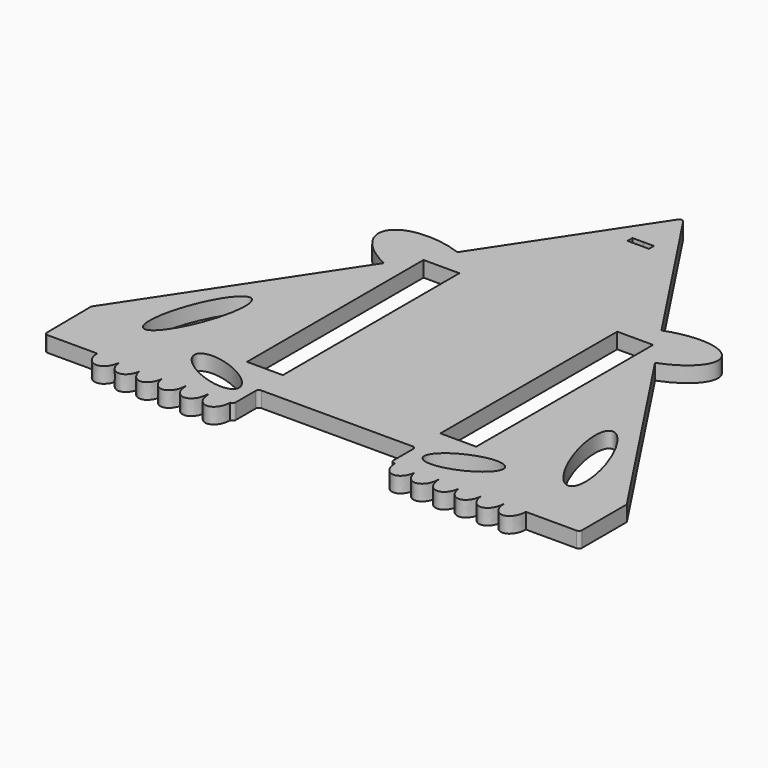
from build123d import *

# Parameters (mm, degrees)
F0_W     = 11.5
F0_H     = 70.714853704
F1_DEPTH = 5


# Not quite as in the source:
# - a feature names something its author has since deleted; it is built from what else it names


with BuildPart() as f1:
    # F0 (on Top) → F1 (new body)
    with BuildSketch(Plane.XY):
        with BuildLine():
            ThreePointArc((-85.7462971022, -48.5098765992), (-85.4499532823, -49.2105923474), (-84.7463458428, -49.5000034571))
            Line((-84.7463458428, -49.5000034571), (-68.8420371116, -49.5000034571))
            Line((-68.8420371116, -49.5000034571), (-61.4353581368, -49.5000034571))
            Line((-61.4353581368, -49.5000034571), (-54.4939316693, -49.5000034571))
            Line((-54.4939316693, -49.5000034571), (-54.4964335859, -50.4300000917))
            add(Edge.make_bspline(
                [(-54.4964335859, -50.4300000917), (-53.9357009598, -54.6615650958), (-50.9232183939, -54.4963216982), (-47.9107358281, -54.3310783007), (-47.5787906349, -50.0505473316)],
                knots=[4.89947782, 4.89947782, 4.89947782, 6.3215634822, 6.3215634822, 7.7436491443, 7.7436491443, 7.7436491443], degree=2, weights=[1, 0.7576817112, 1, 0.7576817112, 1]))
            Line((-47.5787906349, -50.0505473316), (-47.5787906349, -49.5000034571))
            Line((-47.5787906349, -49.5000034571), (-40.6000722349, -49.5000034571))
            Line((-40.6000722349, -49.5000034571), (-40.488735199, -49.5000034571))
            Line((-40.488735199, -49.5000034571), (-33.488735199, -49.5000034571))
            Line((-33.488735199, -49.5000034571), (-33.2292470932, -49.5000034571))
            Line((-33.2292470932, -49.5000034571), (-26.2365209625, -49.5000034571))
            ThreePointArc((-26.2365209625, -49.5000034571), (-26.2328840038, -49.4999968433), (-26.2292470932, -49.4999770021))
            ThreePointArc((-26.2292470932, -49.4999770021), (-25.5268471398, -49.2045338435), (-25.2365209625, -48.5000034571))
            Line((-25.2365209625, -48.5000034571), (-25.2365209625, -40.5000034571))
            ThreePointArc((-25.2365209625, -40.5000034571), (-24.9436277437, -39.7928966759), (-24.2365209625, -39.5000034571))
            Line((-24.2365209625, -39.5000034571), (24.2365209625, -39.5000034571))
            ThreePointArc((24.2365209625, -39.5000034571), (24.9436277437, -39.7928966759), (25.2365209625, -40.5000034571))
            Line((25.2365209625, -40.5000034571), (25.2365209625, -48.5000034571))
            ThreePointArc((25.2365209625, -48.5000034571), (25.5294141813, -49.2071102383), (26.2365209625, -49.5000034571))
            Line((26.2365209625, -49.5000034571), (26.6061850041, -49.5000034571))
            Line((26.6061850041, -49.5000034571), (33.528003484, -49.5000034571))
            Line((33.528003484, -49.5000034571), (33.6061850041, -49.5000034571))
            Line((33.6061850041, -49.5000034571), (40.528003484, -49.5000034571))
            Line((40.528003484, -49.5000034571), (40.6009402275, -49.5000034571))
            Line((40.6009402275, -49.5000034571), (47.5243214667, -49.5000034571))
            Line((47.5243214667, -49.5000034571), (47.6009402275, -49.5000034571))
            Line((47.6009402275, -49.5000034571), (54.5002851784, -49.5000034571))
            Line((54.5002851784, -49.5000034571), (54.5243214667, -49.5000034571))
            Line((54.5243214667, -49.5000034571), (61.5002851784, -49.5000034571))
            Line((61.5002851784, -49.5000034571), (61.5318711996, -49.5000034571))
            Line((61.5318711996, -49.5000034571), (68.5318711996, -49.5000034571))
            Line((68.5318711996, -49.5000034571), (84.7365209625, -49.5000034571))
            ThreePointArc((84.7365209625, -49.5000034571), (85.4436277437, -49.2071102383), (85.7365209625, -48.5000034571))
            Line((85.7365209625, -48.5000034571), (85.7365209625, -30.5649004877))
            Line((85.7365209625, -30.5649004877), (43.3442490508, 33.7225185076))
            Line((43.3442490508, 33.7225185076), (43.3179996887, 33.7225187957))
            add(Edge.make_bspline(
                [(43.3179996887, 33.7225187957), (58.9620766824, 39.6368972474), (54.1362258759, 47.0005661719), (49.3103750694, 54.3642350964), (33.6645006532, 48.4525992955)],
                knots=[1.7240567735, 1.7240567735, 1.7240567735, 3.2946668718, 3.2946668718, 4.86527697, 4.86527697, 4.86527697], degree=2, weights=[1, 0.7071726199, 1, 0.7071726199, 1]))
            Line((33.6645006532, 48.4525992955), (33.6018878615, 48.4967032242))
            Line((33.6018878615, 48.4967032242), (0.951977139, 98.0099375029))
            ThreePointArc((0.951977139, 98.0099375029), (0.1182843378, 98.4594332204), (-0.7164311162, 98.0118394339))
            Line((-0.7164311162, 98.0118394339), (-32.7268251846, 49.708416028))
            add(Edge.make_bspline(
                [(-32.7268251846, 49.708416028), (-48.7950217032, 55.5805403021), (-53.7532185506, 48.0986617244), (-58.7114153979, 40.6167831466), (-43.4232254677, 33.5676352963)],
                knots=[1.511873297, 1.511873297, 1.511873297, 3.0039299939, 3.0039299939, 4.4959866908, 4.4959866908, 4.4959866908], degree=2, weights=[1, 0.7343903226, 1, 0.7343903226, 1]))
            Line((-43.4232254677, 33.5676352963), (-85.9234790375, -30.5649004876))
            Line((-85.9234790375, -30.5649004876), (-85.7462971022, -48.5098765992))
        make_face()
        with BuildLine():
            add(Edge.make_bspline(
                [(-68.1659526923, -31.7135490477), (-60.5147940439, -34.4461020139), (-56.3683340858, -10.7580853655), (-52.2218741276, 12.929931283), (-64.0194927341, -8.0255323992), (-75.8171113406, -28.9809960815), (-68.1659526923, -31.7135490477)],
                knots=[0, 0, 0, 2.0943951024, 2.0943951024, 4.1887902048, 4.1887902048, 6.2831853072, 6.2831853072, 6.2831853072], degree=2, weights=[1, 0.5, 1, 0.5, 1, 0.5, 1]))
        make_face(mode=Mode.SUBTRACT)
        with BuildLine():
            add(Edge.make_bspline(
                [(-49.2456242242, -34.0520180762), (-52.2540837889, -40.9714753387), (-36.0812831751, -43.8893859564), (-19.9084825613, -46.8072965741), (-33.0728236104, -36.9699286939), (-46.2371646594, -27.1325608136), (-49.2456242242, -34.0520180762)],
                knots=[0, 0, 0, 2.0943951024, 2.0943951024, 4.1887902048, 4.1887902048, 6.2831853072, 6.2831853072, 6.2831853072], degree=2, weights=[1, 0.5, 1, 0.5, 1, 0.5, 1]))
        make_face(mode=Mode.SUBTRACT)
        with Locations((-30.9865209625, 5.7290308177)):
            Rectangle(F0_W, F0_H, mode=Mode.SUBTRACT)
        with BuildLine():
            add(Edge.make_bspline(
                [(49.4799129665, -34.0520180762), (46.4714534017, -27.1325608136), (33.3071123527, -36.9699286939), (20.1427713037, -46.8072965741), (36.3155719175, -43.8893859564), (52.4883725313, -40.9714753387), (49.4799129665, -34.0520180762)],
                knots=[0, 0, 0, 2.0943951024, 2.0943951024, 4.1887902048, 4.1887902048, 6.2831853072, 6.2831853072, 6.2831853072], degree=2, weights=[1, 0.5, 1, 0.5, 1, 0.5, 1]))
        make_face(mode=Mode.SUBTRACT)
        with BuildLine():
            add(Edge.make_bspline(
                [(68.4002414346, -31.7135490477), (76.0514000829, -28.9809960815), (64.2537814764, -8.0255323992), (52.4561628699, 12.929931283), (56.6026228281, -10.7580853655), (60.7490827862, -34.4461020139), (68.4002414346, -31.7135490477)],
                knots=[0, 0, 0, 2.0943951024, 2.0943951024, 4.1887902048, 4.1887902048, 6.2831853072, 6.2831853072, 6.2831853072], degree=2, weights=[1, 0.5, 1, 0.5, 1, 0.5, 1]))
        make_face(mode=Mode.SUBTRACT)
        Polygon((36.7681543864, -29.6869881133), (25.2681690006, -29.6686543549), (25.3809054394, 41.0461094846), (36.8808908252, 41.0277757262), align=None, mode=Mode.SUBTRACT)
        with BuildLine():
            Line((-33.5298201198, 48.4967032242), (-32.7268251846, 49.708416028))
            add(Edge.make_bspline(
                [(-31.3512903, 49.1735135083), (-32.0315452267, 49.454325887), (-32.7268251846, 49.708416028)],
                knots=[1.4319341267, 1.4319341267, 1.4319341267, 1.511873297, 1.511873297, 1.511873297], degree=2, weights=[1, 0.9992013225, 1]))
            Line((-31.3512903, 49.1735135083), (-33.5298201198, 48.4967032242))
        make_face(mode=Mode.SUBTRACT)
        Polygon((-3.3304034732, 81.0417085886), (-3.3304034732, 83.0417085886), (0, 83.0417085886), (0.211303281, 83.0415401544), (3.541702522, 83.0362306925), (3.5385140423, 81.0362332341), (0.208110569, 81.0388879667), (0, 81.0390538559), align=None, mode=Mode.SUBTRACT)
        with BuildLine():
            Line((-61.4353581368, -49.5000034571), (-68.8420371116, -49.5000034571))
            add(Edge.make_bspline(
                [(-68.8420371116, -49.5000034571), (-68.8420371116, -54.5000034571), (-65.1386976242, -54.5000034571), (-61.4353581368, -54.5000034571), (-61.4353581368, -49.5000034571)],
                knots=[4.7123889804, 4.7123889804, 4.7123889804, 6.2831853072, 6.2831853072, 7.853981634, 7.853981634, 7.853981634], degree=2, weights=[1, 0.7071067812, 1, 0.7071067812, 1]))
        make_face()
        with BuildLine():
            Line((-26.2365209625, -49.5000034571), (-33.2292470932, -49.5000034571))
            add(Edge.make_bspline(
                [(-33.2292470932, -49.5000034571), (-33.2292470932, -54.5000166846), (-29.729237834, -54.5000034571), (-26.2292285747, -54.4999902295), (-26.2292470932, -49.4999770021)],
                knots=[4.7123889804, 4.7123889804, 4.7123889804, 6.2831879527, 6.2831879527, 7.853986925, 7.853986925, 7.853986925], degree=2, weights=[1, 0.7071058459, 1, 0.7071058459, 1]))
            ThreePointArc((-26.2292470932, -49.4999770021), (-26.2328840038, -49.4999968433), (-26.2365209625, -49.5000034571))
        make_face()
        with BuildLine():
            Line((-33.488735199, -49.5000034571), (-40.488735199, -49.5000034571))
            add(Edge.make_bspline(
                [(-40.488735199, -49.5000034571), (-40.488735199, -54.5000034571), (-36.988735199, -54.5000034571), (-33.488735199, -54.5000034571), (-33.488735199, -49.5000034571)],
                knots=[4.7123889804, 4.7123889804, 4.7123889804, 6.2831853072, 6.2831853072, 7.853981634, 7.853981634, 7.853981634], degree=2, weights=[1, 0.7071067812, 1, 0.7071067812, 1]))
        make_face()
        with BuildLine():
            add(Edge.make_bspline(
                [(61.5318711996, -49.5000034571), (61.5318711996, -54.5000034571), (65.0318711996, -54.5000034571), (68.5318711996, -54.5000034571), (68.5318711996, -49.5000034571)],
                knots=[4.7123889804, 4.7123889804, 4.7123889804, 6.2831853072, 6.2831853072, 7.853981634, 7.853981634, 7.853981634], degree=2, weights=[1, 0.7071067812, 1, 0.7071067812, 1]))
            Line((68.5318711996, -49.5000034571), (61.5318711996, -49.5000034571))
        make_face()
        with BuildLine():
            add(Edge.make_bspline(
                [(54.5123033226, -49.9139998416), (54.7903317418, -54.6944718456), (58.1453084601, -54.4957094189), (61.5002851784, -54.2969469922), (61.5002851784, -49.5000034571)],
                knots=[4.7952831585, 4.7952831585, 4.7952831585, 6.3246323962, 6.3246323962, 7.853981634, 7.853981634, 7.853981634], degree=2, weights=[1, 0.7216076577, 1, 0.7216076577, 1]))
            Line((61.5002851784, -49.5000034571), (54.5243214667, -49.5000034571))
            add(Edge.make_bspline(
                [(54.5123033226, -49.9139998416), (54.5243214667, -49.7073576511), (54.5243214667, -49.5000034571)],
                knots=[1.4879021487, 1.4879021487, 1.4879021487, 1.5707963268, 1.5707963268, 1.5707963268], degree=2, weights=[1, 0.9991411924, 1]))
        make_face()
        with BuildLine():
            Line((-47.5787906349, -49.5000034571), (-47.5787906349, -50.0505473316))
            add(Edge.make_bspline(
                [(-47.5787906349, -50.0505473316), (-47.2141043608, -54.7532841758), (-43.9070882978, -54.4923971), (-40.6000722349, -54.2315100241), (-40.6000722349, -49.5000034571)],
                knots=[4.8227214701, 4.8227214701, 4.8227214701, 6.338351552, 6.338351552, 7.853981634, 7.853981634, 7.853981634], degree=2, weights=[1, 0.7263395445, 1, 0.7263395445, 1]))
            Line((-40.6000722349, -49.5000034571), (-47.5787906349, -49.5000034571))
        make_face()
        with BuildLine():
            add(Edge.make_bspline(
                [(47.5626308471, -50.2377579849), (48.0226120838, -54.6424992613), (51.1383967745, -54.4973470012), (54.2541814653, -54.3521947411), (54.5123033226, -49.9139998416)],
                knots=[4.8604805954, 4.8604805954, 4.8604805954, 6.3157840256, 6.3157840256, 7.7710874559, 7.7710874559, 7.7710874559], degree=2, weights=[1, 0.7467383462, 1, 0.7467383462, 1]))
            add(Edge.make_bspline(
                [(54.5002851784, -49.5000034571), (54.5002851784, -49.7073576511), (54.5123033226, -49.9139998416)],
                knots=[4.7123889804, 4.7123889804, 4.7123889804, 4.7952831585, 4.7952831585, 4.7952831585], degree=2, weights=[1, 0.9991411924, 1]))
            Line((54.5002851784, -49.5000034571), (47.6009402275, -49.5000034571))
            add(Edge.make_bspline(
                [(47.5626308471, -50.2377579849), (47.6009402275, -49.87091061), (47.6009402275, -49.5000034571)],
                knots=[1.4227047118, 1.4227047118, 1.4227047118, 1.5707963268, 1.5707963268, 1.5707963268], degree=2, weights=[1, 0.9972598615, 1]))
        make_face()
        with BuildLine():
            Line((-54.4939316693, -49.5000034571), (-61.4353581368, -49.5000034571))
            add(Edge.make_bspline(
                [(-61.4353581368, -49.5000034571), (-61.4353581368, -54.0528687331), (-58.2622863183, -54.4781430088), (-55.0892144997, -54.9034172845), (-54.4964335859, -50.4300000917)],
                knots=[4.7123889804, 4.7123889804, 4.7123889804, 6.1896408874, 6.1896408874, 7.6668927943, 7.6668927943, 7.6668927943], degree=2, weights=[1, 0.7393943643, 1, 0.7393943643, 1]))
            Line((-54.4964335859, -50.4300000917), (-54.4939316693, -49.5000034571))
        make_face()
        with BuildLine():
            add(Edge.make_bspline(
                [(40.6009402275, -49.5000034571), (40.6009402275, -54.1428346415), (43.8420166563, -54.4863027646), (47.0830930851, -54.8297708877), (47.5626308471, -50.2377579849)],
                knots=[4.7123889804, 4.7123889804, 4.7123889804, 6.2091394997, 6.2091394997, 7.705890019, 7.705890019, 7.705890019], degree=2, weights=[1, 0.7327953886, 1, 0.7327953886, 1]))
            add(Edge.make_bspline(
                [(47.5243214667, -49.5000034571), (47.5243214667, -49.87091061), (47.5626308471, -50.2377579849)],
                knots=[4.7123889804, 4.7123889804, 4.7123889804, 4.8604805954, 4.8604805954, 4.8604805954], degree=2, weights=[1, 0.9972598615, 1]))
            Line((47.5243214667, -49.5000034571), (40.6009402275, -49.5000034571))
        make_face()
        with BuildLine():
            Line((33.528003484, -49.5000034571), (26.6061850041, -49.5000034571))
            add(Edge.make_bspline(
                [(26.6061850041, -49.5000034571), (26.6061850041, -54.1393314863), (29.8446341867, -54.4860229258), (33.0830833693, -54.8327143653), (33.5670942441, -50.24520201)],
                knots=[4.7123889804, 4.7123889804, 4.7123889804, 6.2083867743, 6.2083867743, 7.7043845683, 7.7043845683, 7.7043845683], degree=2, weights=[1, 0.7330514324, 1, 0.7330514324, 1]))
            add(Edge.make_bspline(
                [(33.528003484, -49.5000034571), (33.528003484, -49.8746951598), (33.5670942441, -50.24520201)],
                knots=[4.7123889804, 4.7123889804, 4.7123889804, 4.8619860461, 4.8619860461, 4.8619860461], degree=2, weights=[1, 0.9972038937, 1]))
        make_face()
        with BuildLine():
            add(Edge.make_bspline(
                [(33.5670942441, -50.24520201), (33.6061850041, -49.8746951598), (33.6061850041, -49.5000034571)],
                knots=[1.4211992611, 1.4211992611, 1.4211992611, 1.5707963268, 1.5707963268, 1.5707963268], degree=2, weights=[1, 0.9972038937, 1]))
            add(Edge.make_bspline(
                [(33.5670942441, -50.24520201), (34.0511051188, -54.8327143653), (37.2895543014, -54.4860229258), (40.528003484, -54.1393314863), (40.528003484, -49.5000034571)],
                knots=[4.8619860461, 4.8619860461, 4.8619860461, 6.35798384, 6.35798384, 7.853981634, 7.853981634, 7.853981634], degree=2, weights=[1, 0.7330514324, 1, 0.7330514324, 1]))
            Line((40.528003484, -49.5000034571), (33.6061850041, -49.5000034571))
        make_face()
        with BuildLine():
            add(Edge.make_bspline(
                [(-31.3512903, 49.1735135083), (-32.0315452267, 49.454325887), (-32.7268251846, 49.708416028)],
                knots=[1.4319341267, 1.4319341267, 1.4319341267, 1.511873297, 1.511873297, 1.511873297], degree=2, weights=[1, 0.9992013225, 1]))
            Line((-32.7268251846, 49.708416028), (-33.5298201198, 48.4967032242))
            Line((-33.5298201198, 48.4967032242), (-31.3512903, 49.1735135083))
        make_face()
        with BuildLine():
            Line((33.6061850041, -49.5000034571), (33.528003484, -49.5000034571))
            add(Edge.make_bspline(
                [(33.528003484, -49.5000034571), (33.528003484, -49.8746951598), (33.5670942441, -50.24520201)],
                knots=[4.7123889804, 4.7123889804, 4.7123889804, 4.8619860461, 4.8619860461, 4.8619860461], degree=2, weights=[1, 0.9972038937, 1]))
            add(Edge.make_bspline(
                [(33.5670942441, -50.24520201), (33.6061850041, -49.8746951598), (33.6061850041, -49.5000034571)],
                knots=[1.4211992611, 1.4211992611, 1.4211992611, 1.5707963268, 1.5707963268, 1.5707963268], degree=2, weights=[1, 0.9972038937, 1]))
        make_face()
        with BuildLine():
            add(Edge.make_bspline(
                [(47.5243214667, -49.5000034571), (47.5243214667, -49.87091061), (47.5626308471, -50.2377579849)],
                knots=[4.7123889804, 4.7123889804, 4.7123889804, 4.8604805954, 4.8604805954, 4.8604805954], degree=2, weights=[1, 0.9972598615, 1]))
            add(Edge.make_bspline(
                [(47.5626308471, -50.2377579849), (47.6009402275, -49.87091061), (47.6009402275, -49.5000034571)],
                knots=[1.4227047118, 1.4227047118, 1.4227047118, 1.5707963268, 1.5707963268, 1.5707963268], degree=2, weights=[1, 0.9972598615, 1]))
            Line((47.6009402275, -49.5000034571), (47.5243214667, -49.5000034571))
        make_face()
        with BuildLine():
            add(Edge.make_bspline(
                [(54.5123033226, -49.9139998416), (54.5243214667, -49.7073576511), (54.5243214667, -49.5000034571)],
                knots=[1.4879021487, 1.4879021487, 1.4879021487, 1.5707963268, 1.5707963268, 1.5707963268], degree=2, weights=[1, 0.9991411924, 1]))
            Line((54.5243214667, -49.5000034571), (54.5002851784, -49.5000034571))
            add(Edge.make_bspline(
                [(54.5002851784, -49.5000034571), (54.5002851784, -49.7073576511), (54.5123033226, -49.9139998416)],
                knots=[4.7123889804, 4.7123889804, 4.7123889804, 4.7952831585, 4.7952831585, 4.7952831585], degree=2, weights=[1, 0.9991411924, 1]))
        make_face()
    extrude(amount=F1_DEPTH)


solid = f1.part
